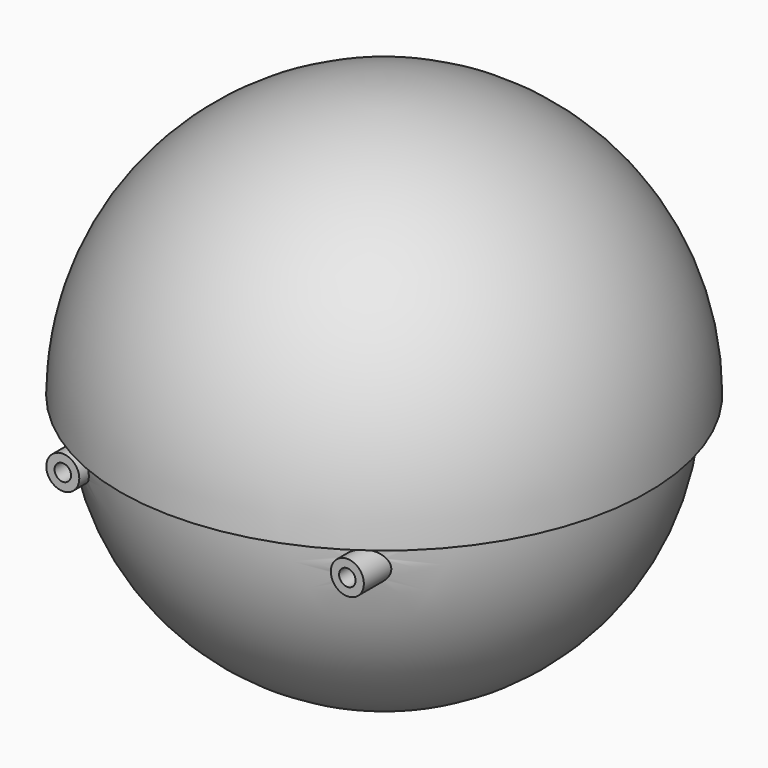
from build123d import *

# Parameters (mm, degrees)
F4_R     = 5
F4_R_2   = 2.5
F5_DEPTH = 67.6


# Not quite as in the source:
# - the program builds the solid bodies; features that only make, move or delete a surface that nothing else refers to are left out


with BuildPart() as f1:
    # F0 (on Front) → F1 (revolve)
    with BuildSketch(Plane.XZ):
        with BuildLine():
            Line((0, -75), (0, 75))
            ThreePointArc((0, 75), (-75, 0), (0, -75))
        make_face()
    revolve(axis=Axis((0, 0, 4.8243552446), (0, 0, 1)))

    # F4 (on Front) → F5 (join)
    with BuildSketch(Plane.XZ):
        with BuildLine():
            ThreePointArc((47.91594401, -7.3852874339), (42.91594401, -2.3852874339), (37.91594401, -7.3852874339))
            ThreePointArc((37.91594401, -7.3852874339), (42.91594401, -12.3852874339), (47.91594401, -7.3852874339))
        make_face()
        with BuildLine():
            ThreePointArc((45.41594401, -7.3852874339), (42.91594401, -9.8852874339), (40.41594401, -7.3852874339))
            ThreePointArc((40.41594401, -7.3852874339), (42.91594401, -4.8852874339), (45.41594401, -7.3852874339))
        make_face(mode=Mode.SUBTRACT)
        with Locations((-43.3072112501, -7.3852874339)):
            Circle(F4_R)
        with Locations((-43.3072112501, -7.3852874339)):
            Circle(F4_R_2, mode=Mode.SUBTRACT)
    extrude(amount=F5_DEPTH)


with BuildPart() as f3:
    # F2 (on Front) → F3 (revolve)
    with BuildSketch(Plane.XZ):
        with BuildLine():
            Line((0, 0), (0, 80))
            ThreePointArc((0, 80), (-56.5685424949, 56.5685424949), (-80, 0))
            Line((-80, 0), (0, 0))
        make_face()
    revolve(axis=Axis((0, 0, -0.3961585462), (0, 0, 1)))


solid = Compound([f1.part, f3.part])
